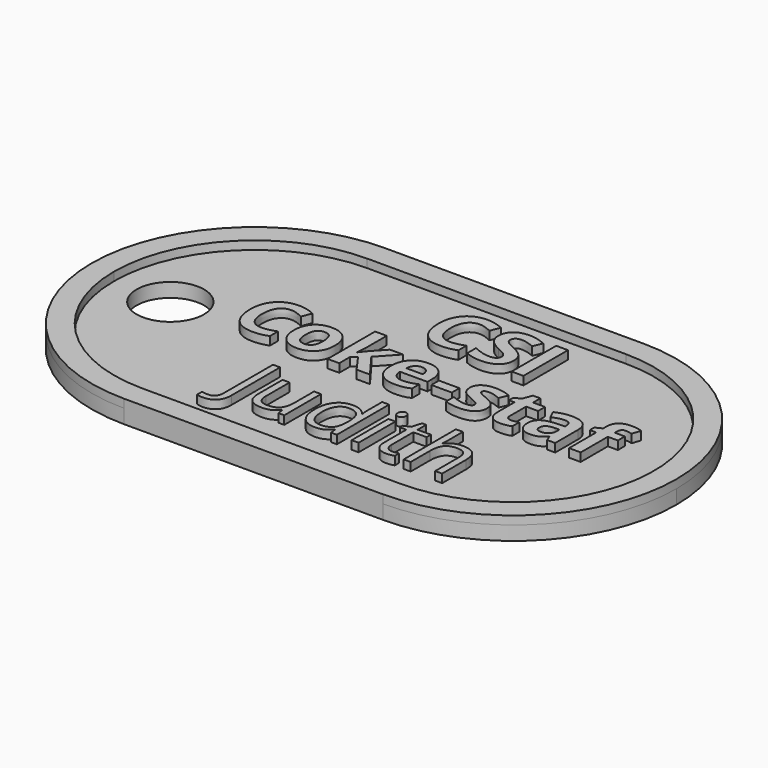
from build123d import *

# Parameters (mm, degrees)
F0_R           = 3
F1_DEPTH       = 1.25
F2_TEXT_SIZE   = 6.9444444444
F3_DEPTH       = 0.75
F2_TEXT_SIZE_2 = 7.6388888889
F4_DEPTH       = 0.75


# Not quite as in the source:
# - a feature names something its author has since deleted; it is built from what else it names
# - Text() gives the source's letters only with a copy of the font that has no kerning and outlines rounded to 1/6400 em; it was checked with that copy


with BuildPart() as f1:
    # F0 (on Top) → F1 (new body)
    with BuildSketch(Plane.XY):
        with BuildLine():
            Line((-11.5, -14.5), (11.5, -14.5))
            ThreePointArc((11.5, -14.5), (21.7530483272, -10.2530483272), (26, 0))
            ThreePointArc((26, 0), (21.7530483272, 10.2530483272), (11.5, 14.5))
            Line((11.5, 14.5), (-11.5, 14.5))
            ThreePointArc((-11.5, 14.5), (-21.7530483272, 10.2530483272), (-26, 0))
            ThreePointArc((-26, 0), (-21.7530483272, -10.2530483272), (-11.5, -14.5))
        make_face()
        with Locations((-19, 0)):
            Circle(F0_R, mode=Mode.SUBTRACT)
    extrude(amount=F1_DEPTH)

    # F2 (on face) → F3 (join)
    with BuildSketch(Plane.XY.offset(1.25)):
        with BuildLine():
            ThreePointArc((-11.5, 14.5), (-26, 0), (-11.5, -14.5))
            Line((-11.5, -14.5), (11.5, -14.5))
            ThreePointArc((11.5, -14.5), (26, 0), (11.5, 14.5))
            Line((11.5, 14.5), (-11.5, 14.5))
        make_face()
        with BuildLine():
            ThreePointArc((11.5, 12.5), (17.7988361106, 10.7969747454), (22.3813399058, 6.1519461844))
            ThreePointArc((22.3813399058, 6.1519461844), (22.2969747454, -6.2988361106), (11.5, -12.5))
            Line((11.5, -12.5), (-11.5, -12.5))
            ThreePointArc((-11.5, -12.5), (-20.3388347648, -8.8388347648), (-24, 0))
            ThreePointArc((-24, 0), (-20.3388347648, 8.8388347648), (-11.5, 12.5))
            Line((-11.5, 12.5), (11.5, 12.5))
        make_face(mode=Mode.SUBTRACT)
        with Locations((-1.9281684028, 5.5)):
            Text('CSI', F2_TEXT_SIZE, font='Open Sans', font_style=FontStyle.BOLD, text_align=(TextAlign.LEFT, TextAlign.BOTTOM))
    extrude(amount=F3_DEPTH)

    # F2 (on face) → F4 (join)
    with BuildSketch(Plane.XY.offset(1.25)):
        with Locations((-13.4809027778, -1)):
            Text('Coke-staf', F2_TEXT_SIZE, font='Open Sans', font_style=FontStyle.BOLD, text_align=(TextAlign.LEFT, TextAlign.BOTTOM))
        with Locations((-7.3423936632, -9.5)):
            Text('Judith', F2_TEXT_SIZE_2, font='Open Sans', text_align=(TextAlign.LEFT, TextAlign.BOTTOM))
    extrude(amount=F4_DEPTH)


solid = f1.part
